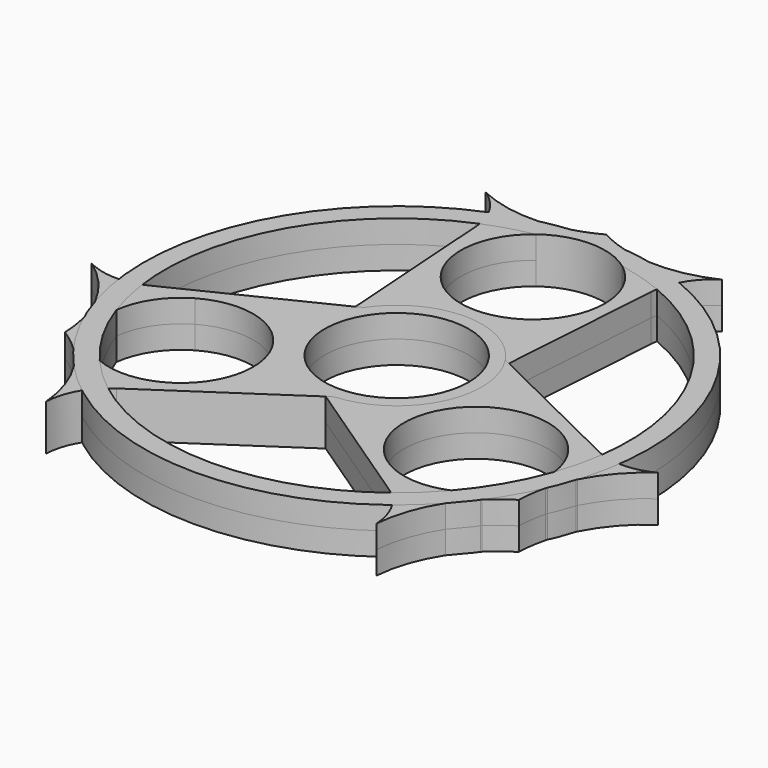
from build123d import *

# Parameters (mm, degrees)
F0_R     = 11
F1_DEPTH = 3.5
F2_COUNT = 3
F3_DEPTH = 3.5


# Not quite as in the source:
# - a feature names something its author has since deleted; it is built from what else it names


with BuildPart() as f1:
    # F0 (on Top) → F1 (new body, symmetric)
    with BuildSketch(Plane.XY):
        with BuildLine():
            ThreePointArc((-11.6552832564, 5.7579833461), (-2.9564605246, -12.6593578497), (13, 0))
            ThreePointArc((13, 0), (12.6593578497, 2.9564605246), (11.6552832564, 5.7579833461))
            ThreePointArc((11.6552832564, 5.7579833461), (0, 13), (-11.6552832564, 5.7579833461))
        make_face()
        Circle(F0_R, mode=Mode.SUBTRACT)
        with BuildLine():
            ThreePointArc((6.588450361, 34.8086503984), (10.1152274328, 33.9519070848), (13.5358418257, 32.7388272054))
            ThreePointArc((13.5358418257, 32.7388272054), (13.9193492029, 34.2721592783), (14.5396613024, 35.7259123706))
            ThreePointArc((14.5396613024, 35.7259123706), (11.535183757, 36.8060063195), (8.4516711937, 37.6339184717))
            ThreePointArc((8.4516711937, 37.6339184717), (6.236572222, 37.8729152879), (4.0617997142, 38.356803159))
            ThreePointArc((4.0617997142, 38.356803159), (0, 38.5712660604), (-4.0617997142, 38.356803159))
            ThreePointArc((-4.0617997142, 38.356803159), (-6.236572222, 37.8729152879), (-8.4516711937, 37.6339184717))
            ThreePointArc((-8.4516711937, 37.6339184717), (-11.535183757, 36.8060063195), (-14.5396613024, 35.7259123706))
            ThreePointArc((-14.5396613024, 35.7259123706), (-13.9193492029, 34.2721592783), (-13.5358418257, 32.7388272054))
            ThreePointArc((-13.5358418257, 32.7388272054), (-10.1152274328, 33.9519070848), (-6.588450361, 34.8086503984))
            ThreePointArc((-6.588450361, 34.8086503984), (0, 37), (6.588450361, 34.8086503984))
        make_face()
        with BuildLine():
            ThreePointArc((-11.6552832564, 5.7579833461), (0, 13), (11.6552832564, 5.7579833461))
            Line((11.6552832564, 5.7579833461), (13.4213995188, 31.7642390728))
            ThreePointArc((13.4213995188, 31.7642390728), (13.4666591176, 32.2529377406), (13.5358418257, 32.7388272054))
            ThreePointArc((13.5358418257, 32.7388272054), (10.1152274328, 33.9519070848), (6.588450361, 34.8086503984))
            ThreePointArc((6.588450361, 34.8086503984), (9.835470349, 30.9258017636), (11, 26))
            ThreePointArc((11, 26), (-4.9258017636, 16.164529651), (-6.588450361, 34.8086503984))
            ThreePointArc((-6.588450361, 34.8086503984), (-10.1152274328, 33.9519070848), (-13.5358418257, 32.7388272054))
            ThreePointArc((-13.5358418257, 32.7388272054), (-13.4666591176, 32.2529377406), (-13.4213995188, 31.7642390728))
            Line((-13.4213995188, 31.7642390728), (-11.6552832564, 5.7579833461))
        make_face()
        with BuildLine():
            ThreePointArc((6.588450361, 34.8086503984), (10.1152274328, 33.9519070848), (13.5358418257, 32.7388272054))
            ThreePointArc((13.5358418257, 32.7388272054), (13.9193492029, 34.2721592783), (14.5396613024, 35.7259123706))
            ThreePointArc((14.5396613024, 35.7259123706), (11.535183757, 36.8060063195), (8.4516711937, 37.6339184717))
            ThreePointArc((8.4516711937, 37.6339184717), (6.236572222, 37.8729152879), (4.0617997142, 38.356803159))
            ThreePointArc((4.0617997142, 38.356803159), (0, 38.5712660604), (-4.0617997142, 38.356803159))
            ThreePointArc((-4.0617997142, 38.356803159), (-6.236572222, 37.8729152879), (-8.4516711937, 37.6339184717))
            ThreePointArc((-8.4516711937, 37.6339184717), (-11.535183757, 36.8060063195), (-14.5396613024, 35.7259123706))
            ThreePointArc((-14.5396613024, 35.7259123706), (-13.9193492029, 34.2721592783), (-13.5358418257, 32.7388272054))
            ThreePointArc((-13.5358418257, 32.7388272054), (-10.1152274328, 33.9519070848), (-6.588450361, 34.8086503984))
            ThreePointArc((-6.588450361, 34.8086503984), (0, 37), (6.588450361, 34.8086503984))
        make_face()
        with BuildLine():
            ThreePointArc((-18.032298954, 39.5249784371), (-16.0366928239, 37.8546254734), (-14.5396613024, 35.7259123706))
            ThreePointArc((-14.5396613024, 35.7259123706), (-11.535183757, 36.8060063195), (-8.4516711937, 37.6339184717))
            ThreePointArc((-8.4516711937, 37.6339184717), (-13.3591775388, 37.9857193268), (-18.032298954, 39.5249784371))
        make_face()
        with BuildLine():
            ThreePointArc((-4.0617997142, 38.356803159), (0, 38.5712660604), (4.0617997142, 38.356803159))
            ThreePointArc((4.0617997142, 38.356803159), (1.985765235, 39.0668338169), (0, 40))
            ThreePointArc((0, 40), (-1.985765235, 39.0668338169), (-4.0617997142, 38.356803159))
        make_face()
        with BuildLine():
            ThreePointArc((8.4516711937, 37.6339184717), (11.535183757, 36.8060063195), (14.5396613024, 35.7259123706))
            ThreePointArc((14.5396613024, 35.7259123706), (16.0366928239, 37.8546254734), (18.032298954, 39.5249784371))
            ThreePointArc((18.032298954, 39.5249784371), (13.3591775388, 37.9857193268), (8.4516711937, 37.6339184717))
        make_face()
    extrude(amount=F1_DEPTH, both=True)


with BuildPart() as f2_1:
    # F2: instance of F1
    add(f1.part.rotate(Axis((0, 0, 0), (0, 0, -1)), 1 * 360 / F2_COUNT))


with BuildPart() as f2_2:
    # F2: instance of F1
    add(f1.part.rotate(Axis((0, 0, 0), (0, 0, -1)), 2 * 360 / F2_COUNT))


with BuildPart() as f3:
    # F0 (on Top) → F3 (new body, symmetric)
    with BuildSketch(Plane.XY):
        with BuildLine():
            ThreePointArc((6.588450361, 34.8086503984), (10.1152274328, 33.9519070848), (13.5358418257, 32.7388272054))
            ThreePointArc((13.5358418257, 32.7388272054), (13.9193492029, 34.2721592783), (14.5396613024, 35.7259123706))
            ThreePointArc((14.5396613024, 35.7259123706), (11.535183757, 36.8060063195), (8.4516711937, 37.6339184717))
            ThreePointArc((8.4516711937, 37.6339184717), (6.236572222, 37.8729152879), (4.0617997142, 38.356803159))
            ThreePointArc((4.0617997142, 38.356803159), (0, 38.5712660604), (-4.0617997142, 38.356803159))
            ThreePointArc((-4.0617997142, 38.356803159), (-6.236572222, 37.8729152879), (-8.4516711937, 37.6339184717))
            ThreePointArc((-8.4516711937, 37.6339184717), (-11.535183757, 36.8060063195), (-14.5396613024, 35.7259123706))
            ThreePointArc((-14.5396613024, 35.7259123706), (-13.9193492029, 34.2721592783), (-13.5358418257, 32.7388272054))
            ThreePointArc((-13.5358418257, 32.7388272054), (-10.1152274328, 33.9519070848), (-6.588450361, 34.8086503984))
            ThreePointArc((-6.588450361, 34.8086503984), (0, 37), (6.588450361, 34.8086503984))
        make_face()
        with BuildLine():
            ThreePointArc((14.5396613024, 35.7259123706), (13.9193492029, 34.2721592783), (13.5358418257, 32.7388272054))
            ThreePointArc((13.5358418257, 32.7388272054), (29.4497859848, 19.6916207094), (35.4266823272, 0))
            ThreePointArc((35.4266823272, 0), (-19.6916207094, -29.4497859848), (-13.5358418257, 32.7388272054))
            ThreePointArc((-13.5358418257, 32.7388272054), (-13.9193492029, 34.2721592783), (-14.5396613024, 35.7259123706))
            ThreePointArc((-14.5396613024, 35.7259123706), (-21.5282305471, -32.0043411901), (38.5712660604, 0))
            ThreePointArc((38.5712660604, 0), (32.0043411901, 21.5282305471), (14.5396613024, 35.7259123706))
        make_face()
        with BuildLine():
            ThreePointArc((8.4516711937, 37.6339184717), (11.535183757, 36.8060063195), (14.5396613024, 35.7259123706))
            ThreePointArc((14.5396613024, 35.7259123706), (16.0366928239, 37.8546254734), (18.032298954, 39.5249784371))
            ThreePointArc((18.032298954, 39.5249784371), (13.3591775388, 37.9857193268), (8.4516711937, 37.6339184717))
        make_face()
        with BuildLine():
            ThreePointArc((-18.032298954, 39.5249784371), (-16.0366928239, 37.8546254734), (-14.5396613024, 35.7259123706))
            ThreePointArc((-14.5396613024, 35.7259123706), (-11.535183757, 36.8060063195), (-8.4516711937, 37.6339184717))
            ThreePointArc((-8.4516711937, 37.6339184717), (-13.3591775388, 37.9857193268), (-18.032298954, 39.5249784371))
        make_face()
        with BuildLine():
            ThreePointArc((4.0617997142, 38.356803159), (6.236572222, 37.8729152879), (8.4516711937, 37.6339184717))
            ThreePointArc((8.4516711937, 37.6339184717), (6.2671667529, 38.0587071035), (4.0617997142, 38.356803159))
        make_face()
        with BuildLine():
            ThreePointArc((-4.0617997142, 38.356803159), (-6.2671667529, 38.0587071035), (-8.4516711937, 37.6339184717))
            ThreePointArc((-8.4516711937, 37.6339184717), (-6.236572222, 37.8729152879), (-4.0617997142, 38.356803159))
        make_face()
        with BuildLine():
            ThreePointArc((-4.0617997142, 38.356803159), (0, 38.5712660604), (4.0617997142, 38.356803159))
            ThreePointArc((4.0617997142, 38.356803159), (1.985765235, 39.0668338169), (0, 40))
            ThreePointArc((0, 40), (-1.985765235, 39.0668338169), (-4.0617997142, 38.356803159))
        make_face()
    extrude(amount=F3_DEPTH, both=True)


solid = Compound([f1.part, f2_1.part, f2_2.part, f3.part])
